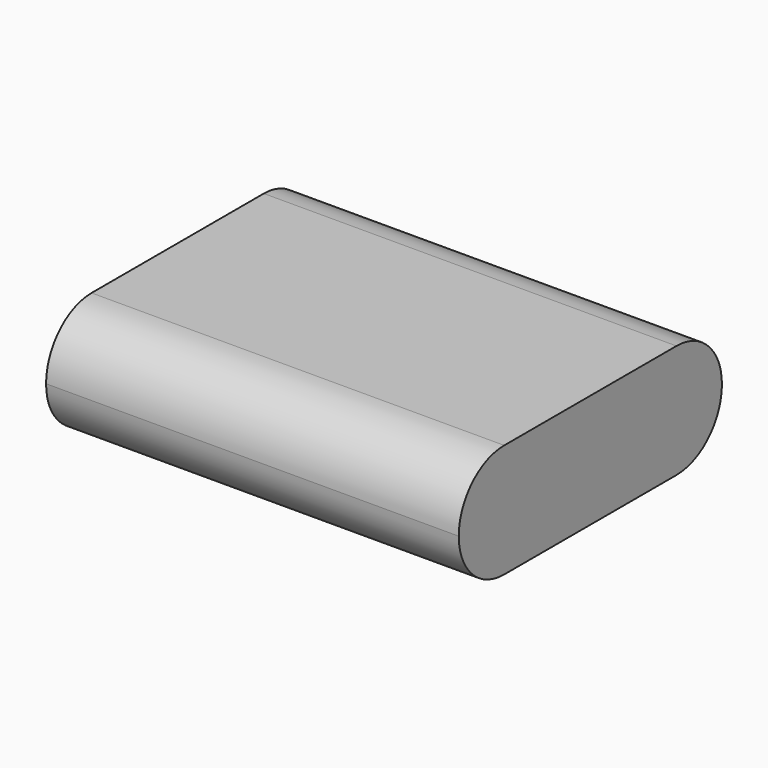
from build123d import *

# Parameters (mm, degrees)
F1_W     = 69
F1_H     = 55
F2_DEPTH = 19
F3_R     = 9.49999


# Not quite as in the source:
# - a fillet or chamfer is up to 0.001 mm smaller than in the source, because OpenCascade refuses the exact size


with BuildPart() as f2:
    # F1 (on Top) → F2 (new body)
    with BuildSketch(Plane.XY):
        with Locations((1.7897747457, 0.8083142097)):
            Rectangle(F1_W, F1_H)
    extrude(amount=F2_DEPTH)

    # F3 (radius 9.5 in the source; OpenCascade refuses exactly that, so slightly less here)
    f3_edges = [f2.edges().sort_by_distance(p)[0] for p in [
        (1.789775, -26.691686, 19),
        (1.789775, -26.691686, 0),
        (1.789775, 28.308314, 19),
        (1.789775, 28.308314, 0),
    ]]
    fillet(f3_edges, radius=F3_R)


solid = f2.part
